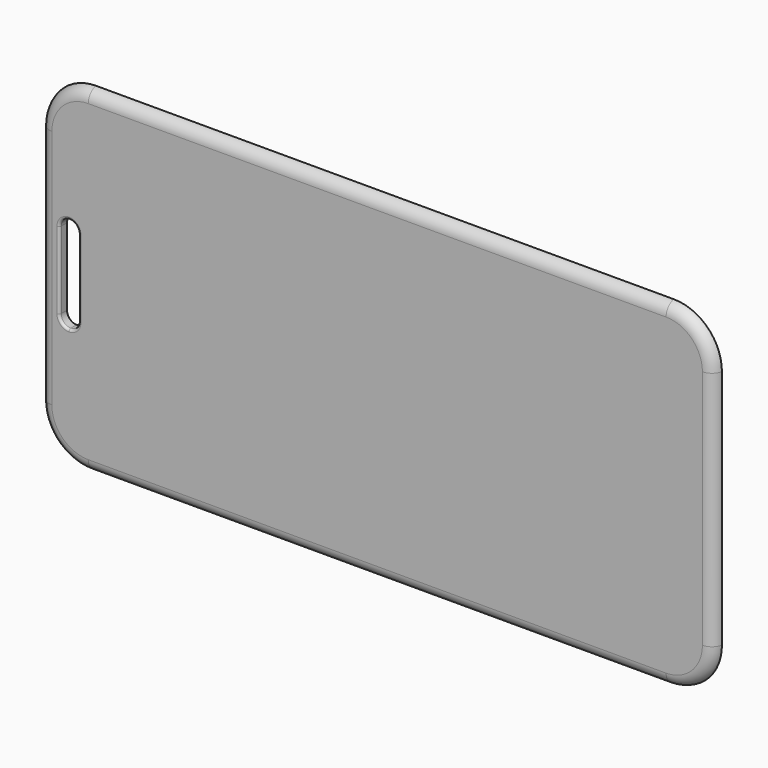
from build123d import *

# Parameters (mm, degrees)
F1_DEPTH     = 2
F3_DEPTH     = 25
F4_T1_DEPTH  = 50
F4_T3_DEPTH  = 120
F4_T6_ANGLE  = 90
F4_T8_ANGLE  = 90
F4_T10_ANGLE = 90
F4_T12_ANGLE = 90
F5_R         = 0.5


# Not quite as in the source:
# - a fillet or chamfer that OpenCascade refuses, or shapes differently, is made with other operations: its cross-section is extruded or revolved along the edge and cut away or added


with BuildPart() as f1:
    # F0 (on Front) → F1 (new body)
    with BuildSketch(Plane.XZ):
        with BuildLine():
            ThreePointArc((70, 25), (67.0710678119, 32.0710678119), (60, 35))
            Line((60, 35), (-60, 35))
            ThreePointArc((-60, 35), (-67.0710678119, 32.0710678119), (-70, 25))
            Line((-70, 25), (-70, -25))
            ThreePointArc((-70, -25), (-67.0710678119, -32.0710678119), (-60, -35))
            Line((-60, -35), (60, -35))
            ThreePointArc((60, -35), (67.0710678119, -32.0710678119), (70, -25))
            Line((70, -25), (70, 25))
        make_face()
    extrude(amount=F1_DEPTH)

    # F2 (on Front) → F3 (cut)
    with BuildSketch(Plane.XZ):
        with BuildLine():
            Line((-62, -8), (-62, 8))
            ThreePointArc((-62, 8), (-62.5857864376, 9.4142135624), (-64, 10))
            ThreePointArc((-64, 10), (-65.4142135624, 9.4142135624), (-66, 8))
            Line((-66, 8), (-66, -8))
            ThreePointArc((-66, -8), (-65.4142135624, -9.4142135624), (-64, -10))
            ThreePointArc((-64, -10), (-62.5857864376, -9.4142135624), (-62, -8))
        make_face()
    extrude(amount=F3_DEPTH, mode=Mode.SUBTRACT)

    # F4: fillet of radius 2.5 on 1 edges, made by hand

    # F4_s2 → F4_t1 (cut)
    with BuildSketch(Plane.XY.offset(-25)):
        with BuildLine():
            ThreePointArc((-67.5505102572, -2), (-69.1316490873, -1.4364916731), (-70, 0))
            Line((-70, 0), (-70, -2))
            Line((-70, -2), (-67.5505102572, -2))
        make_face()
        with BuildLine():
            ThreePointArc((70, 0), (69.1316490873, -1.4364916731), (67.5505102572, -2))
            Line((67.5505102572, -2), (70, -2))
            Line((70, -2), (70, 0))
        make_face()
    extrude(amount=F4_T1_DEPTH, mode=Mode.SUBTRACT)

    # F4_s4 → F4_t3 (cut)
    with BuildSketch(Plane.YZ.offset(-60)):
        with BuildLine():
            ThreePointArc((-2, -32.5505102572), (-1.4364916731, -34.1316490873), (0, -35))
            Line((0, -35), (-2, -35))
            Line((-2, -35), (-2, -32.5505102572))
        make_face()
        with BuildLine():
            ThreePointArc((0, 35), (-1.4364916731, 34.1316490873), (-2, 32.5505102572))
            Line((-2, 32.5505102572), (-2, 35))
            Line((-2, 35), (0, 35))
        make_face()
    extrude(amount=F4_T3_DEPTH, mode=Mode.SUBTRACT)

    # F4_s5 → F4_t6 (revolve, cut)
    with BuildSketch(Plane.XY.offset(-25)):
        with BuildLine():
            ThreePointArc((-67.5505102572, -2), (-69.1316490873, -1.4364916731), (-70, 0))
            Line((-70, 0), (-70, -2))
            Line((-70, -2), (-67.5505102572, -2))
        make_face()
    revolve(axis=Axis((-60, -2, -25), (0, -1, 0)), revolution_arc=F4_T6_ANGLE, mode=Mode.SUBTRACT)

    # F4_s7 → F4_t8 (revolve, cut)
    with BuildSketch(Plane.YZ.offset(60)):
        with BuildLine():
            ThreePointArc((-2, -32.5505102572), (-1.4364916731, -34.1316490873), (0, -35))
            Line((0, -35), (-2, -35))
            Line((-2, -35), (-2, -32.5505102572))
        make_face()
    revolve(axis=Axis((60, -2, -25), (0, -1, 0)), revolution_arc=F4_T8_ANGLE, mode=Mode.SUBTRACT)

    # F4_s9 → F4_t10 (revolve, cut)
    with BuildSketch(Plane.XY.offset(25)):
        with BuildLine():
            ThreePointArc((70, 0), (69.1316490873, -1.4364916731), (67.5505102572, -2))
            Line((67.5505102572, -2), (70, -2))
            Line((70, -2), (70, 0))
        make_face()
    revolve(axis=Axis((60, -2, 25), (0, -1, 0)), revolution_arc=F4_T10_ANGLE, mode=Mode.SUBTRACT)

    # F4_s11 → F4_t12 (revolve, cut)
    with BuildSketch(Plane.YZ.offset(-60)):
        with BuildLine():
            ThreePointArc((-2, 32.5505102572), (-1.4364916731, 34.1316490873), (0, 35))
            Line((0, 35), (-2, 35))
            Line((-2, 35), (-2, 32.5505102572))
        make_face()
    revolve(axis=Axis((-60, -2, 25), (0, -1, 0)), revolution_arc=F4_T12_ANGLE, mode=Mode.SUBTRACT)

    # F5
    f5_edges = [f1.edges().sort_by_distance(p)[0] for p in [
        (-62, -2, 0),
        (-64, -2, 10),
        (-66, -2, 0),
        (-64, -2, -10),
    ]]
    fillet(f5_edges, radius=F5_R)


solid = f1.part
